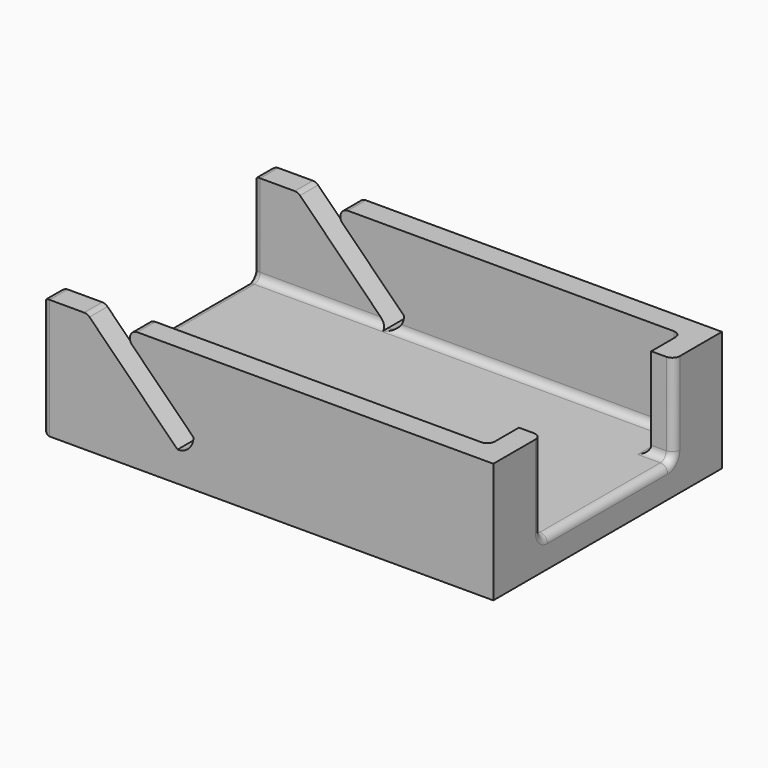
from build123d import *

# Parameters (mm, degrees)
F1_DEPTH     = 20.32
F2_W         = 34.29
F2_H         = 20.32
F3_DEPTH     = 15.24
F4_DEPTH     = 38.1
F6_DEPTH     = 76.2
F7_W         = 27.94
F7_H         = 15.24
F8_DEPTH     = 25.4
F9_T1_DEPTH  = 3.81
F9_T3_DEPTH  = 5.08
F9_T5_DEPTH  = 5.08
F9_T7_DEPTH  = 13.97
F9_S11_W     = 1.2954
F9_S11_H     = 1.2954
F9_T12_DEPTH = 1.2954
F9_S17_W     = 1.2954
F9_S17_H     = 1.2954
F9_T18_DEPTH = 1.2954
F9_T24_DEPTH = 48.26
F9_S25_R     = 2.6940768363
F9_T26_DEPTH = 26
F9_T30_DEPTH = 22.86
F9_T35_DEPTH = 22.86
F9_T40_DEPTH = 48.26
F9_S41_R     = 2.6940768363
F9_T42_DEPTH = 26
F9_T47_DEPTH = 6.985
F9_T51_DEPTH = 8.255
F9_T58_DEPTH = 6.985
F9_T62_DEPTH = 8.255
F9_T65_DEPTH = 25.4
F9_T67_DEPTH = 38.1
F9_T69_DEPTH = 19.1402561211
F9_T71_DEPTH = 6.4402561211
F9_T73_DEPTH = 19.1402561211
F9_T75_DEPTH = 6.4402561211
F9_T77_DEPTH = 54.61
F9_T79_DEPTH = 26.67
F9_T81_DEPTH = 10.16
F9_T83_DEPTH = 17.145
F9_T85_DEPTH = 10.16
F9_T88_ANGLE = 90
F9_T90_ANGLE = 90
F9_T92_ANGLE = 90
F9_T94_ANGLE = 90


# Not quite as in the source:
# - a fillet or chamfer that OpenCascade refuses, or shapes differently, is made with other operations: its cross-section is extruded or revolved along the edge and cut away or added


with BuildPart() as f1:
    # F0 (on Top) → F1 (new body)
    with BuildSketch(Plane.XY):
        Polygon((0, 24.13), (0, 0), (0, -24.13), (38.1, -24.13), (38.1, 24.13), align=None)
    extrude(amount=F1_DEPTH)

    # F2 (on face) → F3 (cut)
    with BuildSketch(Plane.XY.offset(20.32)):
        with Locations((17.145, 10.16)):
            Rectangle(F2_W, F2_H)
        with Locations((17.145, -10.16)):
            Rectangle(F2_W, F2_H)
    extrude(amount=-F3_DEPTH, mode=Mode.SUBTRACT)

    # F4 (add): a face of the model
    f4_faces = [f1.faces().sort_by_distance(p)[0] for p in [
        (0, 0, 0.5236344145),
    ]]
    extrude(f4_faces, amount=F4_DEPTH)

    # F5 (on face) → F6 (cut)
    with BuildSketch(Plane.XZ.offset(24.13)):
        with BuildLine():
            Line((-25.0918463274, 20.32), (-30.48, 20.32))
            Line((-30.48, 20.32), (-15.24, 5.08))
            ThreePointArc((-15.24, 5.08), (-13.335, 5.8690768363), (-12.5459231637, 7.7740768363))
            Line((-12.5459231637, 7.7740768363), (-25.0918463274, 20.32))
        make_face()
    extrude(amount=-F6_DEPTH, mode=Mode.SUBTRACT)

    # F7 (on face) → F8 (cut)
    with BuildSketch(Plane.YZ.offset(38.1)):
        with Locations((0, 12.7)):
            Rectangle(F7_W, F7_H)
    extrude(amount=-F8_DEPTH, mode=Mode.SUBTRACT)

    # F9: fillet of radius 1.27 on 25 edges, made by hand

    # F9_s2 → F9_t1 (join)
    with BuildSketch(Plane.YZ.offset(34.29)):
        with BuildLine():
            ThreePointArc((-12.7, 5.08), (-13.5980256121, 5.4519743879), (-13.97, 6.35))
            Line((-13.97, 6.35), (-13.97, 5.08))
            Line((-13.97, 5.08), (-12.7, 5.08))
        make_face()
        with BuildLine():
            ThreePointArc((13.97, 6.35), (13.5980256121, 5.4519743879), (12.7, 5.08))
            Line((12.7, 5.08), (13.97, 5.08))
            Line((13.97, 5.08), (13.97, 6.35))
        make_face()
    extrude(amount=F9_T1_DEPTH)

    # F9_s4 → F9_t3 (join)
    with BuildSketch(Plane.XZ.offset(13.97)):
        with BuildLine():
            ThreePointArc((33.02, 5.08), (33.9180256121, 5.4519743879), (34.29, 6.35))
            Line((34.29, 6.35), (34.29, 5.08))
            Line((34.29, 5.08), (33.02, 5.08))
        make_face()
    extrude(amount=F9_T3_DEPTH)

    # F9_s6 → F9_t5 (join)
    with BuildSketch(Plane.XZ.offset(-19.05)):
        with BuildLine():
            ThreePointArc((33.02, 5.08), (33.9180256121, 5.4519743879), (34.29, 6.35))
            Line((34.29, 6.35), (34.29, 5.08))
            Line((34.29, 5.08), (33.02, 5.08))
        make_face()
    extrude(amount=F9_T5_DEPTH)

    # F9_s8 → F9_t7 (join)
    with BuildSketch(Plane.XY.offset(6.35)):
        with BuildLine():
            ThreePointArc((34.29, 19.05), (33.9180256121, 19.9480256121), (33.02, 20.32))
            Line((33.02, 20.32), (34.29, 20.32))
            Line((34.29, 20.32), (34.29, 19.05))
        make_face()
        with BuildLine():
            ThreePointArc((34.29, -19.05), (33.9180256121, -19.9480256121), (33.02, -20.32))
            Line((33.02, -20.32), (34.29, -20.32))
            Line((34.29, -20.32), (34.29, -19.05))
        make_face()
    extrude(amount=F9_T7_DEPTH)


with BuildPart() as f9_tool10:
    # F9_s11 → F9_t12 (new body)
    with BuildSketch(Plane.XZ.offset(19.05)):
        with Locations((33.6677, 5.7023)):
            Rectangle(F9_S11_W, F9_S11_H)
    extrude(amount=F9_T12_DEPTH)

    # F9_s13 → F9_t14 (revolve, cut)
    with BuildSketch(Plane(origin=(33.02, -19.05, 6.35), x_dir=(-0.7071067812, 0, 0.7071067812), z_dir=(0.7071067812, 0, 0.7071067812))):
        with BuildLine():
            ThreePointArc((0, -1.27), (1.27, 0), (0, 1.27))
            Line((0, 1.27), (0, -1.27))
        make_face()
    revolve(axis=Axis((33.02, -19.05, 6.35), (0, -1, 0)), mode=Mode.SUBTRACT)


with BuildPart() as f1_1:
    add(f1.part)

    # F9_t9: union F9_tool10
    add(f9_tool10.part)


with BuildPart() as f9_tool16:
    # F9_s17 → F9_t18 (new body)
    with BuildSketch(Plane.XY.offset(6.35)):
        with Locations((33.6677, 19.6977)):
            Rectangle(F9_S17_W, F9_S17_H)
    extrude(amount=-F9_T18_DEPTH)

    # F9_s19 → F9_t20 (revolve, cut)
    with BuildSketch(Plane(origin=(33.02, 19.05, 6.35), x_dir=(-0.7071067812, -0.7071067812, 0), z_dir=(0.7071067812, -0.7071067812, 0))):
        with BuildLine():
            ThreePointArc((0, -1.27), (1.27, 0), (0, 1.27))
            Line((0, 1.27), (0, -1.27))
        make_face()
    revolve(axis=Axis((33.02, 19.05, 6.35), (0, 0, -1)), mode=Mode.SUBTRACT)


with BuildPart() as f1_2:
    add(f1_1.part)

    # F9_t15: union F9_tool16
    add(f9_tool16.part)


with BuildPart() as f9_tool22:
    # F9_s23 → F9_t24 (new body)
    with BuildSketch(Plane.YZ.offset(33.02)):
        with BuildLine():
            ThreePointArc((-19.05, 5.08), (-19.9480256121, 5.4519743879), (-20.32, 6.35))
            Line((-20.32, 6.35), (-20.32, 5.08))
            Line((-20.32, 5.08), (-19.05, 5.08))
        make_face()
    extrude(amount=-F9_T24_DEPTH)

    # F9_s25 → F9_t26 (cut, symmetric)
    with BuildSketch(Plane.XZ.offset(19.7)):
        with Locations((-15.24, 7.7740768363)):
            Circle(F9_S25_R)
    extrude(amount=F9_T26_DEPTH, both=True, mode=Mode.SUBTRACT)


with BuildPart() as f1_3:
    add(f1_2.part)

    # F9_t21: union F9_tool22
    add(f9_tool22.part)


with BuildPart() as f9_tool28:
    # F9_s29 → F9_t30 (new body)
    with BuildSketch(Plane.YZ.offset(-15.24)):
        with BuildLine():
            ThreePointArc((-19.05, 5.08), (-19.9480256121, 5.4519743879), (-20.32, 6.35))
            Line((-20.32, 6.35), (-20.32, 5.08))
            Line((-20.32, 5.08), (-19.05, 5.08))
        make_face()
    extrude(amount=-F9_T30_DEPTH)

    split(bisect_by=Plane(origin=(-5.08, 0, -5.08), x_dir=(0, 1, 0), z_dir=(-0.7071067812, 0, -0.7071067812)), keep=Keep.TOP)


with BuildPart() as f1_4:
    add(f1_3.part)

    # F9_t27: union F9_tool28
    add(f9_tool28.part)


with BuildPart() as f9_tool33:
    # F9_s34 → F9_t35 (new body)
    with BuildSketch(Plane.YZ.offset(-15.24)):
        with BuildLine():
            ThreePointArc((19.05, 5.08), (19.9480256121, 5.4519743879), (20.32, 6.35))
            Line((20.32, 6.35), (20.32, 5.08))
            Line((20.32, 5.08), (19.05, 5.08))
        make_face()
    extrude(amount=-F9_T35_DEPTH)

    split(bisect_by=Plane(origin=(-5.08, 0, -5.08), x_dir=(0, 1, 0), z_dir=(-0.7071067812, 0, -0.7071067812)), keep=Keep.TOP)


with BuildPart() as f1_5:
    add(f1_4.part)

    # F9_t32: union F9_tool33
    add(f9_tool33.part)


with BuildPart() as f9_tool38:
    # F9_s39 → F9_t40 (new body)
    with BuildSketch(Plane.YZ.offset(33.02)):
        with BuildLine():
            ThreePointArc((19.05, 5.08), (19.9480256121, 5.4519743879), (20.32, 6.35))
            Line((20.32, 6.35), (20.32, 5.08))
            Line((20.32, 5.08), (19.05, 5.08))
        make_face()
    extrude(amount=-F9_T40_DEPTH)

    # F9_s41 → F9_t42 (cut, symmetric)
    with BuildSketch(Plane.XZ.offset(-19.7)):
        with Locations((-15.24, 7.7740768363)):
            Circle(F9_S41_R)
    extrude(amount=F9_T42_DEPTH, both=True, mode=Mode.SUBTRACT)


with BuildPart() as f1_6:
    add(f1_5.part)

    # F9_t37: union F9_tool38
    add(f9_tool38.part)


with BuildPart() as f9_tool45:
    # F9_s46 → F9_t47 (new body)
    with BuildSketch(Plane.YZ.offset(38.1)):
        with BuildLine():
            ThreePointArc((-12.7, 5.08), (-13.5980256121, 5.4519743879), (-13.97, 6.35))
            Line((-13.97, 6.35), (-13.97, 5.08))
            Line((-13.97, 5.08), (-12.7, 5.08))
        make_face()
    extrude(amount=-F9_T47_DEPTH)

    split(bisect_by=Plane.YZ.offset(34.29), keep=Keep.BOTTOM)


with BuildPart() as f9_tool49:
    # F9_s50 → F9_t51 (new body)
    with BuildSketch(Plane.XZ.offset(19.05)):
        with BuildLine():
            ThreePointArc((33.02, 5.08), (33.9180256121, 5.4519743879), (34.29, 6.35))
            Line((34.29, 6.35), (34.29, 5.08))
            Line((34.29, 5.08), (33.02, 5.08))
        make_face()
    extrude(amount=-F9_T51_DEPTH)

    split(bisect_by=Plane.XZ.offset(13.97), keep=Keep.BOTTOM)


with BuildPart() as f9_tool45_1:
    add(f9_tool45.part)

    # F9_t53: intersect F9_tool49
    add(f9_tool49.part, mode=Mode.INTERSECT)


with BuildPart() as f1_7:
    add(f1_6.part)

    # F9_t43: union F9_tool45
    add(f9_tool45_1.part)


with BuildPart() as f9_tool56:
    # F9_s57 → F9_t58 (new body)
    with BuildSketch(Plane.YZ.offset(38.1)):
        with BuildLine():
            ThreePointArc((13.97, 6.35), (13.5980256121, 5.4519743879), (12.7, 5.08))
            Line((12.7, 5.08), (13.97, 5.08))
            Line((13.97, 5.08), (13.97, 6.35))
        make_face()
    extrude(amount=-F9_T58_DEPTH)

    split(bisect_by=Plane.YZ.offset(34.29), keep=Keep.BOTTOM)


with BuildPart() as f9_tool60:
    # F9_s61 → F9_t62 (new body)
    with BuildSketch(Plane.XZ.offset(-10.795)):
        with BuildLine():
            ThreePointArc((33.02, 5.08), (33.9180256121, 5.4519743879), (34.29, 6.35))
            Line((34.29, 6.35), (34.29, 5.08))
            Line((34.29, 5.08), (33.02, 5.08))
        make_face()
    extrude(amount=-F9_T62_DEPTH)

    split(bisect_by=Plane.XZ.offset(-13.97), keep=Keep.TOP)


with BuildPart() as f9_tool56_1:
    add(f9_tool56.part)

    # F9_t64: intersect F9_tool60
    add(f9_tool60.part, mode=Mode.INTERSECT)


with BuildPart() as f1_8:
    add(f1_7.part)

    # F9_t54: union F9_tool56
    add(f9_tool56_1.part)

    # F9_s66 → F9_t65 (cut)
    with BuildSketch(Plane.XZ.offset(-12.7)):
        with BuildLine():
            ThreePointArc((36.83, 5.08), (37.7280256121, 4.7080256121), (38.1, 3.81))
            Line((38.1, 3.81), (38.1, 5.08))
            Line((38.1, 5.08), (36.83, 5.08))
        make_face()
    extrude(amount=F9_T65_DEPTH, mode=Mode.SUBTRACT)

    # F9_s68 → F9_t67 (cut)
    with BuildSketch(Plane.XZ.offset(-19.05)):
        with BuildLine():
            ThreePointArc((-38.1, 3.81), (-37.7280256121, 4.7080256121), (-36.83, 5.08))
            Line((-36.83, 5.08), (-38.1, 5.08))
            Line((-38.1, 5.08), (-38.1, 3.81))
        make_face()
    extrude(amount=F9_T67_DEPTH, mode=Mode.SUBTRACT)

    # F9_s70 → F9_t69 (cut)
    with BuildSketch(Plane.XZ.offset(-31.7951280605)):
        with BuildLine():
            ThreePointArc((-22.9238207153, 18.1519743879), (-23.1991221094, 19.5360079591), (-22.0257951031, 20.32))
            Line((-22.0257951031, 20.32), (-25.0918463274, 20.32))
            Line((-25.0918463274, 20.32), (-22.9238207153, 18.1519743879))
        make_face()
    extrude(amount=F9_T69_DEPTH, mode=Mode.SUBTRACT)

    # F9_s72 → F9_t71 (cut)
    with BuildSketch(Plane.XZ.offset(-25.4451280605)):
        with BuildLine():
            ThreePointArc((-30.1080256121, 19.9480256121), (-30.5200432651, 20.2233270063), (-31.0060512242, 20.32))
            Line((-31.0060512242, 20.32), (-30.48, 20.32))
            Line((-30.48, 20.32), (-30.1080256121, 19.9480256121))
        make_face()
    extrude(amount=F9_T71_DEPTH, mode=Mode.SUBTRACT)

    # F9_s74 → F9_t73 (cut)
    with BuildSketch(Plane.XZ.offset(12.6548719395)):
        with BuildLine():
            ThreePointArc((-22.9238207153, 18.1519743879), (-23.1991221094, 19.5360079591), (-22.0257951031, 20.32))
            Line((-22.0257951031, 20.32), (-25.0918463274, 20.32))
            Line((-25.0918463274, 20.32), (-22.9238207153, 18.1519743879))
        make_face()
    extrude(amount=F9_T73_DEPTH, mode=Mode.SUBTRACT)

    # F9_s76 → F9_t75 (cut)
    with BuildSketch(Plane.XZ.offset(19.0048719395)):
        with BuildLine():
            ThreePointArc((-31.0060512242, 20.32), (-30.5200432651, 20.2233270063), (-30.1080256121, 19.9480256121))
            Line((-30.1080256121, 19.9480256121), (-30.48, 20.32))
            Line((-30.48, 20.32), (-31.0060512242, 20.32))
        make_face()
    extrude(amount=F9_T75_DEPTH, mode=Mode.SUBTRACT)

    # F9_s78 → F9_t77 (cut)
    with BuildSketch(Plane.XZ.offset(-27.305)):
        with BuildLine():
            ThreePointArc((-36.83, 0), (-37.7280256121, 0.3719743879), (-38.1, 1.27))
            Line((-38.1, 1.27), (-38.1, 0))
            Line((-38.1, 0), (-36.83, 0))
        make_face()
    extrude(amount=F9_T77_DEPTH, mode=Mode.SUBTRACT)

    # F9_s80 → F9_t79 (cut)
    with BuildSketch(Plane.XY.offset(-3.175)):
        with BuildLine():
            ThreePointArc((-38.1, -22.86), (-37.7280256121, -23.7580256121), (-36.83, -24.13))
            Line((-36.83, -24.13), (-38.1, -24.13))
            Line((-38.1, -24.13), (-38.1, -22.86))
        make_face()
        with BuildLine():
            ThreePointArc((-38.1, 22.86), (-37.7280256121, 23.7580256121), (-36.83, 24.13))
            Line((-36.83, 24.13), (-38.1, 24.13))
            Line((-38.1, 24.13), (-38.1, 22.86))
        make_face()
    extrude(amount=F9_T79_DEPTH, mode=Mode.SUBTRACT)

    # F9_s82 → F9_t81 (cut)
    with BuildSketch(Plane.XZ.offset(17.145)):
        with BuildLine():
            ThreePointArc((-38.1, 19.05), (-37.7280256121, 19.9480256121), (-36.83, 20.32))
            Line((-36.83, 20.32), (-38.1, 20.32))
            Line((-38.1, 20.32), (-38.1, 19.05))
        make_face()
    extrude(amount=F9_T81_DEPTH, mode=Mode.SUBTRACT)

    # F9_s84 → F9_t83 (cut)
    with BuildSketch(Plane.XY.offset(6.35)):
        with BuildLine():
            ThreePointArc((-38.1, -21.59), (-37.7280256121, -20.6919743879), (-36.83, -20.32))
            Line((-36.83, -20.32), (-38.1, -20.32))
            Line((-38.1, -20.32), (-38.1, -21.59))
        make_face()
        with BuildLine():
            ThreePointArc((-38.1, 21.59), (-37.7280256121, 20.6919743879), (-36.83, 20.32))
            Line((-36.83, 20.32), (-38.1, 20.32))
            Line((-38.1, 20.32), (-38.1, 21.59))
        make_face()
        with BuildLine():
            ThreePointArc((36.83, 13.97), (37.7280256121, 14.3419743879), (38.1, 15.24))
            Line((38.1, 15.24), (38.1, 13.97))
            Line((38.1, 13.97), (36.83, 13.97))
        make_face()
        with BuildLine():
            ThreePointArc((36.83, -13.97), (37.7280256121, -14.3419743879), (38.1, -15.24))
            Line((38.1, -15.24), (38.1, -13.97))
            Line((38.1, -13.97), (36.83, -13.97))
        make_face()
    extrude(amount=F9_T83_DEPTH, mode=Mode.SUBTRACT)

    # F9_s86 → F9_t85 (cut)
    with BuildSketch(Plane.XZ.offset(-27.305)):
        with BuildLine():
            ThreePointArc((-38.1, 19.05), (-37.7280256121, 19.9480256121), (-36.83, 20.32))
            Line((-36.83, 20.32), (-38.1, 20.32))
            Line((-38.1, 20.32), (-38.1, 19.05))
        make_face()
    extrude(amount=F9_T85_DEPTH, mode=Mode.SUBTRACT)

    # F9_s87 → F9_t88 (revolve, cut)
    with BuildSketch(Plane.XZ.offset(12.7)):
        with BuildLine():
            ThreePointArc((36.83, 5.08), (37.7280256121, 4.7080256121), (38.1, 3.81))
            Line((38.1, 3.81), (38.1, 5.08))
            Line((38.1, 5.08), (36.83, 5.08))
        make_face()
    revolve(axis=Axis((38.1, -12.7, 6.35), (-1, 0, 0)), revolution_arc=F9_T88_ANGLE, mode=Mode.SUBTRACT)

    # F9_s89 → F9_t90 (revolve, cut)
    with BuildSketch(Plane.XY.offset(6.35)):
        with BuildLine():
            ThreePointArc((36.83, 13.97), (37.7280256121, 14.3419743879), (38.1, 15.24))
            Line((38.1, 15.24), (38.1, 13.97))
            Line((38.1, 13.97), (36.83, 13.97))
        make_face()
    revolve(axis=Axis((38.1, 12.7, 6.35), (-1, 0, 0)), revolution_arc=F9_T90_ANGLE, mode=Mode.SUBTRACT)

    # F9_s91 → F9_t92 (revolve, cut)
    with BuildSketch(Plane.XZ.offset(-19.05)):
        with BuildLine():
            ThreePointArc((-38.1, 3.81), (-37.7280256121, 4.7080256121), (-36.83, 5.08))
            Line((-36.83, 5.08), (-38.1, 5.08))
            Line((-38.1, 5.08), (-38.1, 3.81))
        make_face()
    revolve(axis=Axis((-38.1, 19.05, 6.35), (1, 0, 0)), revolution_arc=F9_T92_ANGLE, mode=Mode.SUBTRACT)

    # F9_s93 → F9_t94 (revolve, cut)
    with BuildSketch(Plane.XZ.offset(19.05)):
        with BuildLine():
            ThreePointArc((-38.1, 3.81), (-37.7280256121, 4.7080256121), (-36.83, 5.08))
            Line((-36.83, 5.08), (-38.1, 5.08))
            Line((-38.1, 5.08), (-38.1, 3.81))
        make_face()
    revolve(axis=Axis((-38.1, -19.05, 6.35), (-1, 0, 0)), revolution_arc=F9_T94_ANGLE, mode=Mode.SUBTRACT)


solid = f1_8.part
